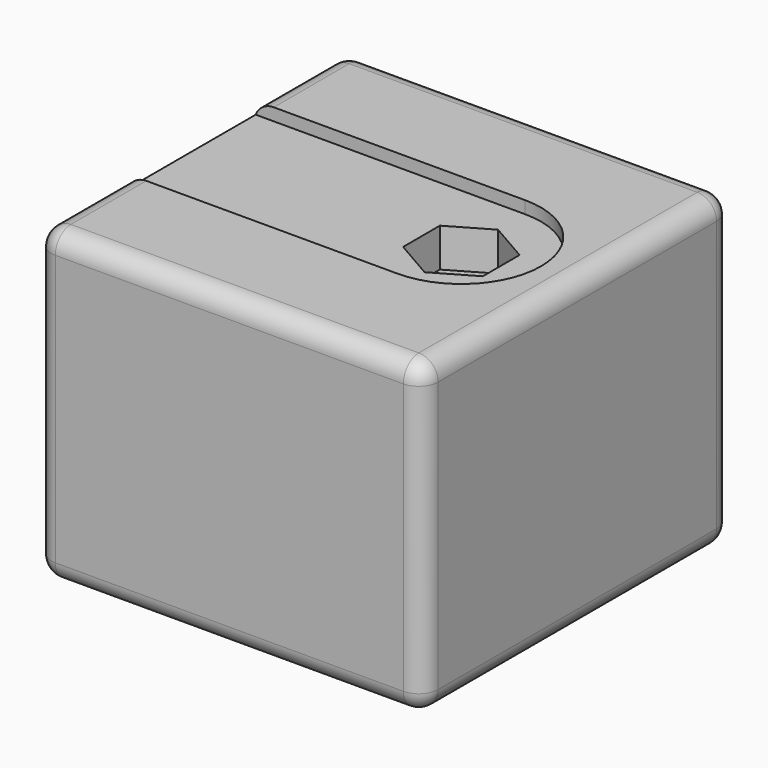
from build123d import *

# Parameters (mm, degrees)
F0_W     = 63.5
F0_H     = 63.5
F1_DEPTH = 50.8
F4_DEPTH = 2.032
F2_W     = 1.5281873676
F2_H     = 5.9584317987
F5_DEPTH = 8.382
F6_F1_R  = 3.175
F6_F2_R  = 3.175
F6_F3_R  = 3.175
F6_F4_R  = 3.175
F6_F5_R  = 3.175


with BuildPart() as f1:
    # F0 (on Top) → F1 (new body)
    with BuildSketch(Plane.XY):
        Rectangle(F0_W, F0_H)
    extrude(amount=F1_DEPTH)

    # F3 (on face) → F4 (cut)
    with BuildSketch(Plane.XY.offset(50.8)):
        with BuildLine():
            Line((-31.75, -13.081), (12.7, -13.081))
            ThreePointArc((12.7, -13.081), (25.781, 0), (12.7, 13.081))
            Line((12.7, 13.081), (-31.75, 13.081))
            Line((-31.75, 13.081), (-31.75, -13.081))
        make_face()
        Polygon((12.7063958977, -7.552316163), (6.1627002943, -3.7816970914), (6.1563043966, 3.7706190716), (12.6936041023, 7.552316163), (19.2372997057, 3.7816970914), (19.2436956034, -3.7706190716), align=None, mode=Mode.SUBTRACT)
    extrude(amount=-F4_DEPTH, mode=Mode.SUBTRACT)

    # F2 (on face) → F5 (cut)
    with BuildSketch(Plane.XY.offset(50.8)):
        with Locations((145.2675004168, 51.4206579864)):
            Rectangle(F2_W, F2_H)
        Polygon((12.6936041023, 7.552316163), (6.1563043966, 3.7706190716), (6.1627002943, -3.7816970914), (12.7063958977, -7.552316163), (19.2436956034, -3.7706190716), (19.2372997057, 3.7816970914), align=None)
    extrude(amount=-F5_DEPTH, mode=Mode.SUBTRACT)

    # F6: fillet of radius 3.175 on 13 edges, made by hand

    # F6_f1
    f6_f1_edges = [f1.edges().sort_by_distance(p)[0] for p in [
        (-31.75, 0, 0),
    ]]
    fillet(f6_f1_edges, radius=F6_F1_R)

    # F6_f2
    f6_f2_edges = [f1.edges().sort_by_distance(p)[0] for p in [
        (-31.75, -31.75, 26.9875),
    ]]
    fillet(f6_f2_edges, radius=F6_F2_R)

    # F6_f3
    f6_f3_edges = [f1.edges().sort_by_distance(p)[0] for p in [
        (-31.75, -20.828, 50.8),
    ]]
    fillet(f6_f3_edges, radius=F6_F3_R)

    # F6_f4
    f6_f4_edges = [f1.edges().sort_by_distance(p)[0] for p in [
        (-31.75, 31.75, 25.4),
    ]]
    fillet(f6_f4_edges, radius=F6_F4_R)

    # F6_f5
    f6_f5_edges = [f1.edges().sort_by_distance(p)[0] for p in [
        (31.75, 0, 0),
    ]]
    fillet(f6_f5_edges, radius=F6_F5_R)


solid = f1.part
